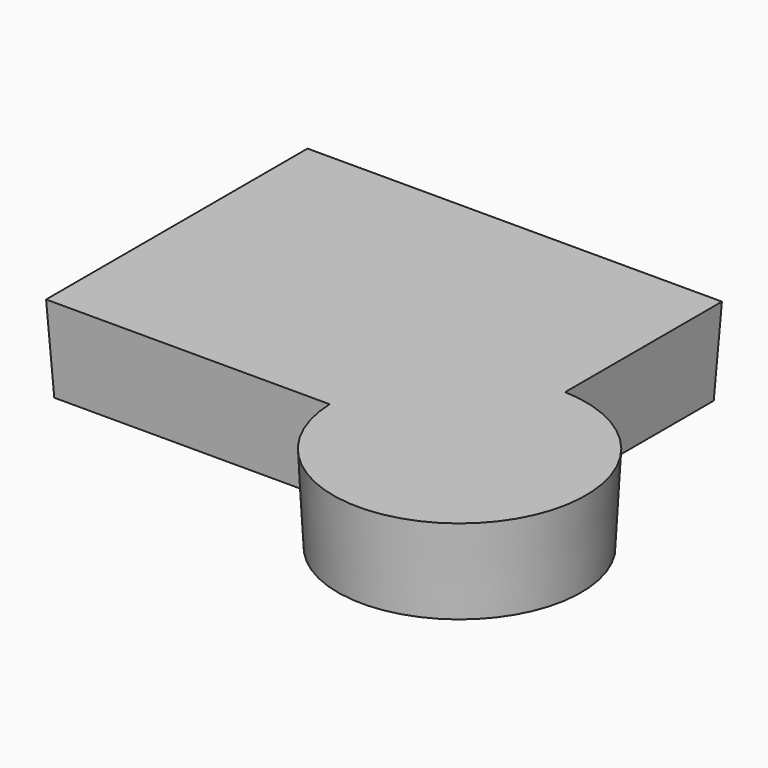
from build123d import *

# Parameters (mm, degrees)
F1_DEPTH               = 25
DRAFT_F1_DRAFTED_ANGLE = -3


# Not quite as in the source:
# - an extrude with a draft is written as a straight extrude whose walls are then drafted


with BuildPart() as f1:
    # F0 (on Top) → F1 (new body)
    with BuildSketch(Plane.XY):
        with BuildLine():
            Line((-92.8765311837, 52.1933399141), (-92.8765311837, -39.2127670348))
            Line((-92.8765311837, -39.2127670348), (-11.3176227796, -39.2127670348))
            ThreePointArc((-11.3176227796, -39.2127670348), (48.4897951039, -63.9858106526), (23.7167514861, -4.1783927691))
            Line((23.7167514861, -4.1783927691), (23.7167514861, 52.1933399141))
            Line((23.7167514861, 52.1933399141), (-92.8765311837, 52.1933399141))
        make_face()
    extrude(amount=F1_DEPTH)

    # draft_F1_drafted
    draft_f1_drafted_walls = [f1.faces().sort_by_distance(p)[0] for p in [
        (23.7167514861, 24.0074735725, 16.6666666667),
        (-34.5798898488, 52.1933399141, 16.6666666667),
        (-92.8765311837, 6.4902864397, 16.6666666667),
        (-52.0970769817, -39.2127670348, 16.6666666667),
        (48.4897951039, -63.9858106526, 16.6666666667),
    ]]
    draft(draft_f1_drafted_walls, neutral_plane=Plane.XY, angle=DRAFT_F1_DRAFTED_ANGLE)


solid = f1.part
